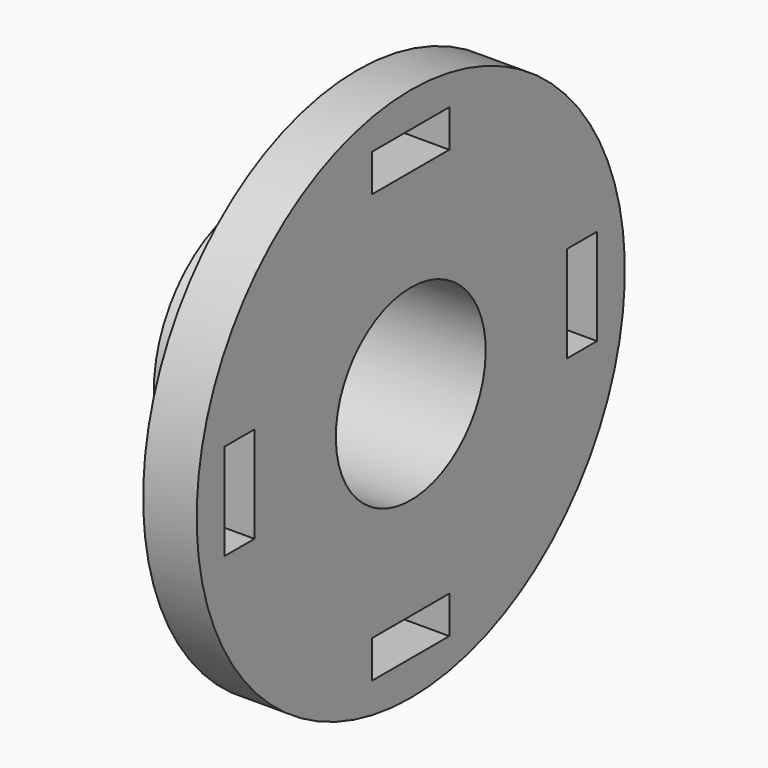
from build123d import *

# Parameters (mm, degrees)
F2_W            = 18
F2_H            = 7
F3_DEPTH        = 30.001
F3_COPIES_COUNT = 4


# Not quite as in the source:
# - a pattern or mirror of a feature is missing from the dataset's text; its kind, count and spacing are read off the source's solid


with BuildPart() as f1:
    # F0 (on Front) → F1 (revolve)
    with BuildSketch(Plane.XZ):
        Polygon((0, 17.5), (0, 50), (-10, 50), (-10, 22.5), (-30, 22.5), (-30, 17.5), align=None)
    revolve(axis=Axis((23.6921556821, 0, 0), (1, 0, 0)))

    # F2 (on face) → F3 (cut, through all)
    with BuildSketch(Plane.YZ):
        with Locations((0, 40)):
            Rectangle(F2_W, F2_H)
    f3 = extrude(amount=-F3_DEPTH, mode=Mode.SUBTRACT)

    # F3_copies: F3 ×4 about axis
    f3_copies_axis = Axis((0, 0, 0), (1, 0, 0))
    for i in range(1, F3_COPIES_COUNT):
        add(f3.rotate(f3_copies_axis, i * 360 / F3_COPIES_COUNT), mode=Mode.SUBTRACT)


solid = f1.part
